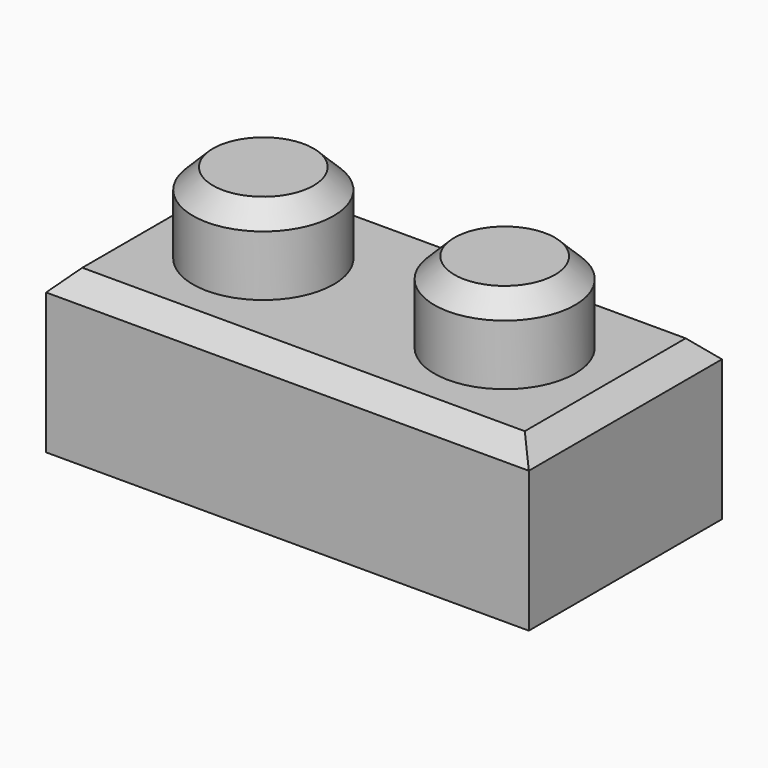
from build123d import *

# Parameters (mm, degrees)
F0_W     = 76.2
F0_H     = 38.1
F1_DEPTH = 25.4
F2_R     = 11.1125
F3_DEPTH = 12.7
F4_SIZE2 = 3.175
F4_SIZE  = 3.175
F5_T     = 7.9375


# Not quite as in the source:
# - a shell that OpenCascade refuses in one call is made with other operations: the cavity is built on its own and cut out


with BuildPart() as f1:
    # F0 (on Top) → F1 (new body)
    with BuildSketch(Plane.XY):
        with Locations((-38.1, 3.6128160983)):
            Rectangle(F0_W, F0_H)
    extrude(amount=F1_DEPTH)

    # F2 (on face) → F3 (join)
    with BuildSketch(Plane.XY.offset(25.4)):
        with Locations((-57.15, 3.6128160983)):
            Circle(F2_R)
        with Locations((-19.05, 3.6128160983)):
            Circle(F2_R)
    extrude(amount=F3_DEPTH)

    # F4
    f4_edges = [f1.edges().sort_by_distance(p)[0] for p in [
        (-68.2625, 3.612816, 38.1),
        (-30.1625, 3.612816, 38.1),
        (-38.1, -15.437184, 25.4),
        (0, 3.612816, 25.4),
        (-38.1, 22.662816, 25.4),
        (-76.2, 3.612816, 25.4),
    ]]
    chamfer(f4_edges, length=F4_SIZE, length2=F4_SIZE2)

    # F5: shell of thickness 7.9375, made by hand


with BuildPart() as f5_core1:
    # F5_t2: copy of F1
    add(f1.part)

    # the walls: a layer under each face that stays
    f5_faces = [f5_core1.faces().sort_by_distance(p)[0] for p in [
        (0, 3.6128160983, 11.1125),
        (-38.1, -15.4371839017, 11.1125),
        (-1.5875, 3.6128160983, 23.8125),
        (-38.1, 22.6628160983, 11.1125),
        (-76.2, 3.6128160983, 11.1125),
        (-38.1, -13.8496839017, 23.8125),
        (-38.1, 3.6128160983, 25.4),
        (-38.1, 21.0753160983, 23.8125),
        (-74.6125, 3.6128160983, 23.8125),
        (-68.2625, 3.6128160983, 30.1625),
        (-30.1625, 3.6128160983, 30.1625),
        (-66.675, 3.6128160983, 36.5125),
        (-28.575, 3.6128160983, 36.5125),
        (-57.15, 3.6128160983, 38.1),
        (-19.05, 3.6128160983, 38.1),
    ]]
    thicken(f5_faces, amount=-F5_T, mode=Mode.SUBTRACT)

    # F5_s3 → F5_t4 (revolve, cut)
    with BuildSketch(Plane.XZ.offset(-3.6128160983)):
        Polygon((-45.958125, 25.479375), (-46.0375, 17.4625), (-53.975, 17.4625), (-53.975, 25.4), align=None)
    revolve(axis=Axis((-57.15, 3.6128160983, 25.4), (0, 0, 1)), mode=Mode.SUBTRACT)

    # F5_s5 → F5_t6 (revolve, cut)
    with BuildSketch(Plane.XZ.offset(-3.6128160983)):
        Polygon((-7.858125, 25.479375), (-7.9375, 17.4625), (-15.875, 17.4625), (-15.875, 25.4), align=None)
    revolve(axis=Axis((-19.05, 3.6128160983, 25.4), (0, 0, 1)), mode=Mode.SUBTRACT)


with BuildPart() as f1_1:
    add(f1.part)

    # what is left inside the walls is the cavity
    f5_cavity = [f5_core1.part.solids().sort_by_distance(p)[0] for p in [
        (-38.1, -0.091351, 0.079375),
    ]]
    add(f5_cavity, mode=Mode.SUBTRACT)


solid = f1_1.part
